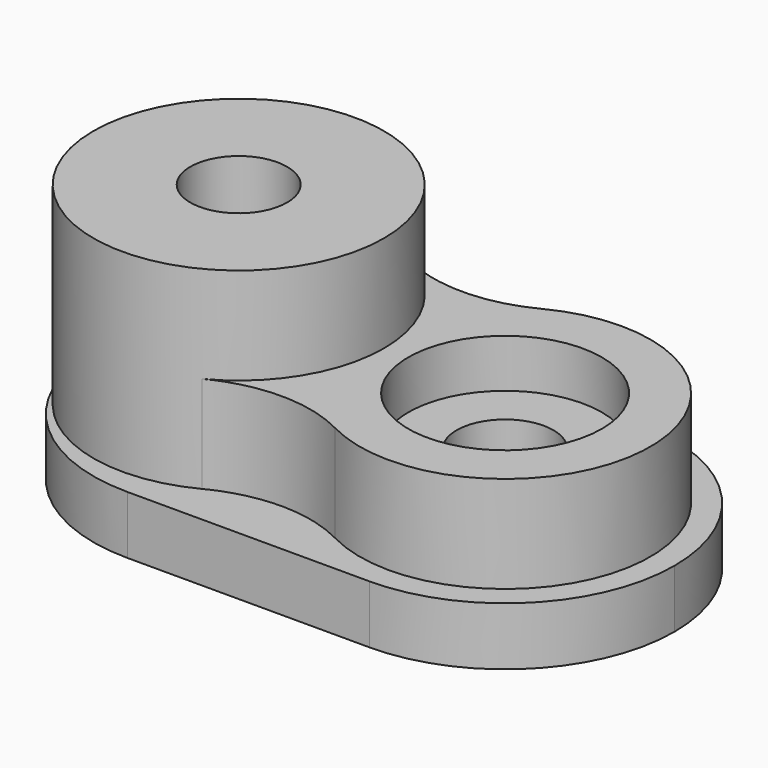
from build123d import *

# Parameters (mm, degrees)
F0_W          = 24
F0_H          = 14
F1_DEPTH      = 2.4
F3_R          = 6
F4_DEPTH      = 8
F5_R          = 6
F6_DEPTH      = 4
F2_R          = 2
F7_DEPTH      = 2.401
F7_DEPTH_BACK = 8.001
F8_R          = 2
F9_DEPTH      = 6.401
F10_R         = 3.5
F11_DEPTH     = 2
F12_R         = 4
F13_DEPTH     = 2
F14_T1_DEPTH  = 37.4
F15_R         = 6


# Not quite as in the source:
# - a fillet or chamfer that OpenCascade refuses, or shapes differently, is made with other operations: its cross-section is extruded or revolved along the edge and cut away or added


with BuildPart() as f1:
    # F0 (on Top) → F1 (new body)
    with BuildSketch(Plane.XY):
        with Locations((-3.2606057666, 7)):
            Rectangle(F0_W, F0_H)
    extrude(amount=F1_DEPTH)

    # F3 (on face) → F4 (join)
    with BuildSketch(Plane.XY.offset(2.4)):
        with Locations((-9.2606057666, 7)):
            Circle(F3_R)
    extrude(amount=F4_DEPTH)

    # F5 (on face) → F6 (join)
    with BuildSketch(Plane.XY.offset(2.4)):
        with Locations((1.7393942334, 7)):
            Circle(F5_R)
    extrude(amount=F6_DEPTH)

    # F2 (on face) → F7 (cut, two sides)
    with BuildSketch(Plane.XY.offset(2.4)) as f7_sk:
        with Locations((-9.2606057666, 7)):
            Circle(F2_R)
    extrude(amount=-F7_DEPTH, mode=Mode.SUBTRACT)
    extrude(f7_sk.sketch, amount=F7_DEPTH_BACK, mode=Mode.SUBTRACT)

    # F8 (on face) → F9 (cut, through all)
    with BuildSketch(Plane.XY.offset(6.4)):
        with Locations((1.7393942334, 7)):
            Circle(F8_R)
    extrude(amount=-F9_DEPTH, mode=Mode.SUBTRACT)

    # F10 (on face) → F11 (cut)
    with BuildSketch(Plane(origin=(0, 0, 0), x_dir=(1, 0, 0), z_dir=(0, 0, -1))):
        with Locations((1.7393942334, -7)):
            Circle(F10_R)
    extrude(amount=-F11_DEPTH, mode=Mode.SUBTRACT)

    # F12 (on face) → F13 (cut)
    with BuildSketch(Plane.XY.offset(6.4)):
        with Locations((1.7393942334, 7)):
            Circle(F12_R)
    extrude(amount=-F13_DEPTH, mode=Mode.SUBTRACT)

    # F14: fillet of radius 7 on 4 edges, made by hand

    # F14_s2 → F14_t1 (cut)
    with BuildSketch(Plane.XY.offset(-17.5)):
        with BuildLine():
            ThreePointArc((-8.2606057666, 14), (-13.2103532349, 11.9497474683), (-15.2606057666, 7))
            Line((-15.2606057666, 7), (-15.2606057666, 14))
            Line((-15.2606057666, 14), (-8.2606057666, 14))
        make_face()
        with BuildLine():
            ThreePointArc((-15.2606057666, 7), (-13.2103532349, 2.0502525317), (-8.2606057666, 0))
            Line((-8.2606057666, 0), (-15.2606057666, 0))
            Line((-15.2606057666, 0), (-15.2606057666, 7))
        make_face()
        with BuildLine():
            ThreePointArc((8.7393942334, 7), (6.6891417017, 2.0502525317), (1.7393942334, 0))
            Line((1.7393942334, 0), (8.7393942334, 0))
            Line((8.7393942334, 0), (8.7393942334, 7))
        make_face()
        with BuildLine():
            ThreePointArc((1.7393942334, 14), (6.6891417017, 11.9497474683), (8.7393942334, 7))
            Line((8.7393942334, 7), (8.7393942334, 14))
            Line((8.7393942334, 14), (1.7393942334, 14))
        make_face()
    extrude(amount=F14_T1_DEPTH, mode=Mode.SUBTRACT)

    # F15
    f15_edges = [f1.edges().sort_by_distance(p)[0] for p in [
        (-3.760606, 4.602084, 4.4),
        (-3.760606, 9.397916, 4.4),
    ]]
    fillet(f15_edges, radius=F15_R)


solid = f1.part
